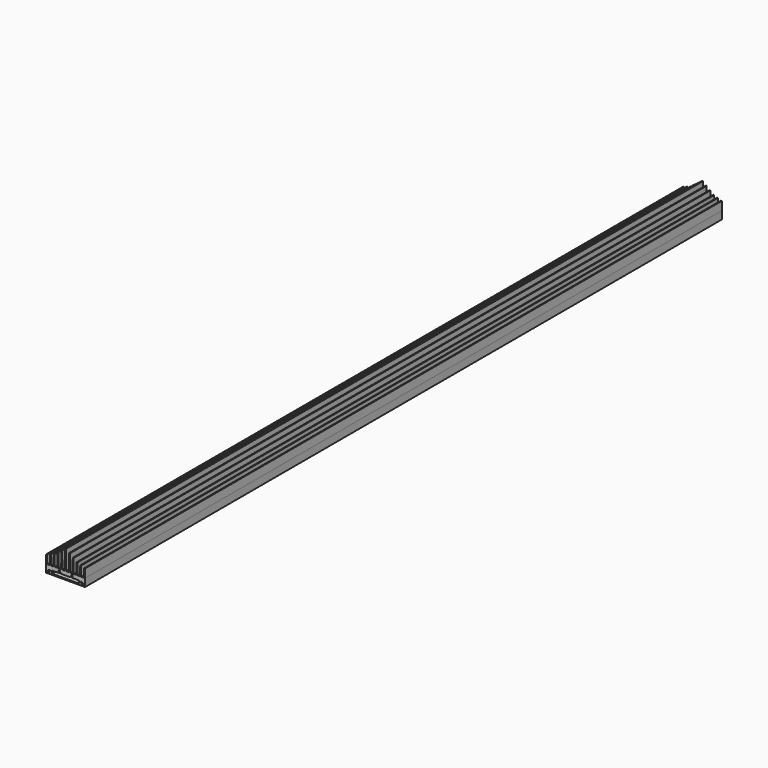
from build123d import *

# Parameters (mm, degrees)
F1_DEPTH = 1420
F3_DEPTH = 1420


with BuildPart() as f1:
    # F0 (on Front) → F1 (new body)
    with BuildSketch(Plane.XZ):
        with BuildLine():
            Line((-32.7227568555, 3.4999999998), (-32.9727568555, 18.4999999998))
            Line((-32.9727568555, 18.4999999998), (-34.4727568555, 18.4999999998))
            Line((-34.4727568555, 18.4999999998), (-34.7227568555, 3.4999999998))
            Line((-34.7227568555, 3.4999999998), (-34.7227568555, -10.5000000002))
            Line((-34.7227568555, -10.5000000002), (-27.5528838745, -10.5000000002))
            Line((-27.5528838745, -10.5000000002), (-27.5528838745, -6.5000000002))
            Line((-27.5528838745, -6.5000000002), (-28.5528838745, -6.5000000002))
            Line((-28.5528838745, -6.5000000002), (-28.5528838745, -8.0000000002))
            Line((-28.5528838745, -8.0000000002), (-32.0528838745, -8.0000000002))
            Line((-32.0528838745, -8.0000000002), (-32.0528838745, -6.0000000002))
            Line((-32.0528838745, -6.0000000002), (-27.7227568555, -3.5000000002))
            Line((-27.7227568555, -3.5000000002), (-27.1091535687, -3.5000000002))
            Line((-27.1091535687, -3.5000000002), (-25.3028838745, -3.5000000002))
            Line((-25.3028838745, -3.5000000002), (-25.3028838745, -8.5000000002))
            Line((-25.3028838745, -8.5000000002), (-23.8028838745, -8.5000000002))
            Line((-23.8028838745, -8.5000000002), (-23.8028838745, -3.5000000002))
            Line((-23.8028838745, -3.5000000002), (-11.2141814145, -3.5000000002))
            Line((-11.2141814145, -3.5000000002), (-12.8211504387, -1.5848888924))
            Line((-12.8211504387, -1.5848888924), (-12.8211504387, 0.3141777723))
            ThreePointArc((-12.8211504387, 0.3141777723), (-11.5711504387, 1.5641777723), (-10.3211504387, 0.3141777723))
            Line((-10.3211504387, 0.3141777723), (-10.3211504387, -0.4358222277))
            Line((-10.3211504387, -0.4358222277), (-7.75, -3.5000000002))
            Line((-7.75, -3.5000000002), (0, -3.5000000002))
            Line((0, -3.5000000002), (0, 38.4999999998))
            Line((0, 38.4999999998), (-0.75, 38.4999999998))
            Line((-0.75, 38.4999999998), (-1, 3.4999999998))
            Line((-1, 3.4999999998), (-5.75, 3.4999999998))
            Line((-5.75, 3.4999999998), (-6, 33.4999999998))
            Line((-6, 33.4999999998), (-7.5, 33.4999999998))
            Line((-7.5, 33.4999999998), (-7.75, 3.4999999998))
            Line((-7.75, 3.4999999998), (-12.6212390675, 3.4999999998))
            Line((-12.6212390675, 3.4999999998), (-12.8712390675, 28.4999999998))
            Line((-12.8712390675, 28.4999999998), (-14.3712390675, 28.4999999998))
            Line((-14.3712390675, 28.4999999998), (-14.6212390675, 3.5015064141))
            Line((-14.6212390675, 3.5015064141), (-19.2384126596, 3.4999999998))
            Line((-19.2384126596, 3.4999999998), (-19.4884126596, 23.4999999998))
            Line((-19.4884126596, 23.4999999998), (-20.9884126596, 23.4999999998))
            Line((-20.9884126596, 23.4999999998), (-21.2384126596, 3.4999999998))
            Line((-21.2384126596, 3.4999999998), (-26, 3.4999999998))
            Line((-26, 3.4999999998), (-26.25, 20.9999999998))
            Line((-26.25, 20.9999999998), (-27.75, 20.9999999998))
            Line((-27.75, 20.9999999998), (-28, 3.4999999998))
            Line((-28, 3.4999999998), (-32.7227568555, 3.4999999998))
        make_face()
    extrude(amount=F1_DEPTH)

    # F4: F1 across face


with BuildPart() as f3:
    # F2 (on face) → F3 (new body)
    with BuildSketch(Plane.XZ.offset(1420)):
        Polygon((-25.3028838745, -8.5000000002), (-25.3028838745, -3.5000000002), (-27.3028838745, -3.5000000002), (-27.3028838745, -10.5000000002), (0, -10.5000000002), (0, -8.5000000002), align=None)
    extrude(amount=-F3_DEPTH)

    # F5: F3 across face


with BuildPart() as f1_1:
    add(f1.part)
    add(f1.part.mirror(Plane(origin=(0, -710, 17.4999999998), x_dir=(0, 1, 0), z_dir=(1, 0, 0))))


with BuildPart() as f3_1:
    add(f3.part)
    add(f3.part.mirror(Plane(origin=(0, -710, -9.5000000002), x_dir=(0, 1, 0), z_dir=(1, 0, 0))))


solid = Compound([f1_1.part, f3_1.part])
